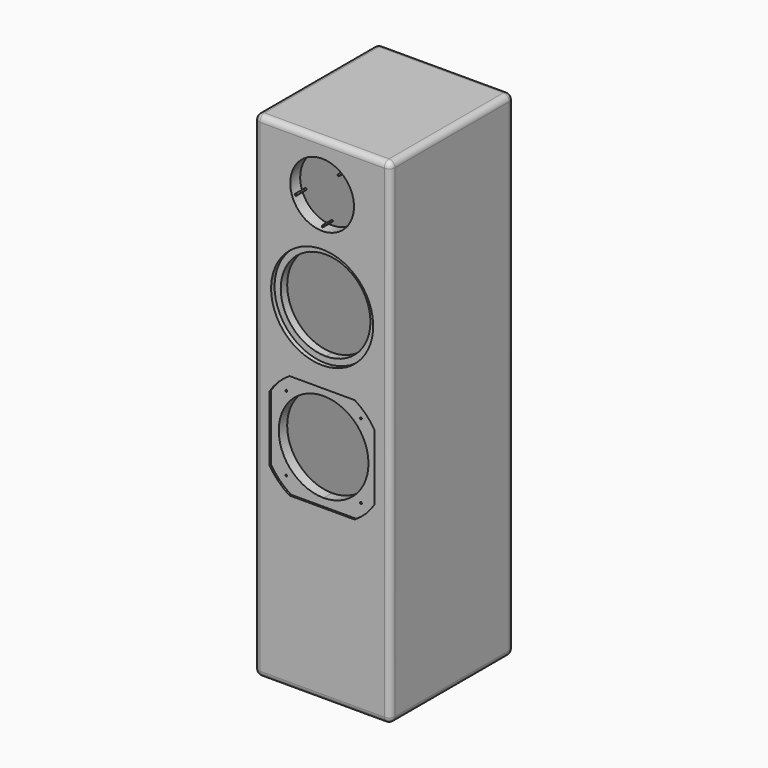
from build123d import *

# Parameters (mm, degrees)
F0_W     = 180
F0_H     = 210
F1_DEPTH = 20
F0_W_2   = 220
F0_H_2   = 250
F2_DEPTH = 800
F3_W     = 180
F3_H     = 210
F4_DEPTH = 20
F5_R     = 1.5
F6_DEPTH = 20
F7_DEPTH = 7
F8_DEPTH = 3
F9_R     = 9.5


with BuildPart() as f1:
    # F0 (on Top) → F1 (new body)
    with BuildSketch(Plane.XY):
        Rectangle(F0_W, F0_H)
    extrude(amount=F1_DEPTH)

    # F0 (on Top) → F2 (join)
    with BuildSketch(Plane.XY):
        Rectangle(F0_W_2, F0_H_2)
        Rectangle(F0_W, F0_H, mode=Mode.SUBTRACT)
    extrude(amount=F2_DEPTH)

    # F3 (on face) → F4 (join)
    with BuildSketch(Plane.XY.offset(800)):
        Rectangle(F3_W, F3_H)
    extrude(amount=-F4_DEPTH)

    # F5 (on face) → F6 (cut)
    with BuildSketch(Plane.XZ.offset(125)):
        with BuildLine():
            ThreePointArc((51.5, 720), (36.4159992311, 756.4159992311), (0, 771.5))
            Line((0, 771.5), (0, 765))
            ThreePointArc((0, 765), (13.1905408693, 763.023361463), (25.2222847872, 757.2670947367))
            ThreePointArc((25.2222847872, 757.2670947367), (26.9019571294, 757.8361628294), (27.9503363532, 756.4057647469))
            ThreePointArc((27.9503363532, 756.4057647469), (27.8730087425, 755.9303667321), (27.6489986565, 755.5039839073))
            ThreePointArc((27.6489986565, 755.5039839073), (40.4302172857, 739.7584799574), (45, 720))
            ThreePointArc((45, 720), (44.5571276947, 713.7021931119), (43.2372279289, 707.5283473019))
            ThreePointArc((43.2372279289, 707.5283473019), (44.0036790141, 706.9859955787), (44.2975432333, 706.0942352531))
            ThreePointArc((44.2975432333, 706.0942352531), (43.6690774316, 704.8734043307), (42.3103057118, 704.6755740541))
            ThreePointArc((42.3103057118, 704.6755740541), (26.4503363532, 683.5942352531), (1.4997916522, 675.025))
            ThreePointArc((1.4997916522, 675.025), (1.4999479121, 675.0125004341), (1.5, 675))
            ThreePointArc((1.5, 675), (1.0606601718, 673.9393398282), (0, 673.5))
            Line((0, 673.5), (0, 668.5))
            ThreePointArc((0, 668.5), (36.4159992311, 683.5840007689), (51.5, 720))
        make_face()
        with BuildLine():
            Line((0, 765), (0, 771.5))
            ThreePointArc((0, 771.5), (-51.5, 720), (0, 668.5))
            Line((0, 668.5), (0, 673.5))
            ThreePointArc((0, 673.5), (-1.0694624818, 673.9482158016), (-1.4997916522, 675.025))
            ThreePointArc((-1.4997916522, 675.025), (-26.4503363532, 683.5942352531), (-42.3103057118, 704.6755740541))
            ThreePointArc((-42.3103057118, 704.6755740541), (-44.2241280077, 705.6307097616), (-43.2372279289, 707.5283473019))
            ThreePointArc((-43.2372279289, 707.5283473019), (-42.7975432333, 733.9057647469), (-27.6489986565, 755.5039839073))
            ThreePointArc((-27.6489986565, 755.5039839073), (-27.3320142316, 757.6192902384), (-25.2222847872, 757.2670947367))
            ThreePointArc((-25.2222847872, 757.2670947367), (-13.1905408693, 763.023361463), (0, 765))
        make_face()
        with BuildLine():
            ThreePointArc((25.2222847872, 757.2670947367), (13.1905408693, 763.023361463), (0, 765))
            Line((0, 765), (0, 760))
            ThreePointArc((0, 760), (28.2842712475, 748.2842712475), (40, 720))
            ThreePointArc((40, 720), (28.2842712475, 691.7157287525), (0, 680))
            Line((0, 680), (0, 676.5))
            ThreePointArc((0, 676.5), (1.0517841984, 676.0694624818), (1.4997916522, 675.025))
            ThreePointArc((1.4997916522, 675.025), (26.4503363532, 683.5942352531), (42.3103057118, 704.6755740541))
            ThreePointArc((42.3103057118, 704.6755740541), (41.3709584588, 706.5577607447), (43.2372279289, 707.5283473019))
            ThreePointArc((43.2372279289, 707.5283473019), (44.5571276947, 713.7021931119), (45, 720))
            ThreePointArc((45, 720), (40.4302172857, 739.7584799574), (27.6489986565, 755.5039839073))
            ThreePointArc((27.6489986565, 755.5039839073), (25.5686584747, 755.1922392553), (25.2222847872, 757.2670947367))
        make_face()
        with BuildLine():
            Line((0, 760), (0, 765))
            ThreePointArc((0, 765), (-13.1905408693, 763.023361463), (-25.2222847872, 757.2670947367))
            ThreePointArc((-25.2222847872, 757.2670947367), (-25.0199382706, 756.8573855231), (-24.9503363532, 756.4057647469))
            ThreePointArc((-24.9503363532, 756.4057647469), (-25.9749383383, 754.9830923575), (-27.6489986565, 755.5039839073))
            ThreePointArc((-27.6489986565, 755.5039839073), (-42.7975432333, 733.9057647469), (-43.2372279289, 707.5283473019))
            ThreePointArc((-43.2372279289, 707.5283473019), (-41.9057829077, 707.3003710339), (-41.2975432333, 706.0942352531))
            ThreePointArc((-41.2975432333, 706.0942352531), (-41.5767123109, 705.2227010548), (-42.3103057118, 704.6755740541))
            ThreePointArc((-42.3103057118, 704.6755740541), (-26.4503363532, 683.5942352531), (-1.4997916522, 675.025))
            ThreePointArc((-1.4997916522, 675.025), (-1.0517841984, 676.0694624818), (0, 676.5))
            Line((0, 676.5), (0, 680))
            ThreePointArc((0, 680), (-40, 720), (0, 760))
        make_face()
        with BuildLine():
            ThreePointArc((40, 720), (28.2842712475, 748.2842712475), (0, 760))
            Line((0, 760), (0, 680))
            ThreePointArc((0, 680), (28.2842712475, 691.7157287525), (40, 720))
        make_face()
        with BuildLine():
            Line((0, 680), (0, 760))
            ThreePointArc((0, 760), (-40, 720), (0, 680))
        make_face()
        with BuildLine():
            ThreePointArc((-24.9503363532, 756.4057647469), (-25.0199382706, 756.8573855231), (-25.2222847872, 757.2670947367))
            ThreePointArc((-25.2222847872, 757.2670947367), (-26.4503363532, 756.4057647469), (-27.6489986565, 755.5039839073))
            ThreePointArc((-27.6489986565, 755.5039839073), (-25.9749383383, 754.9830923575), (-24.9503363532, 756.4057647469))
        make_face()
        with BuildLine():
            ThreePointArc((-27.6489986565, 755.5039839073), (-26.4503363532, 756.4057647469), (-25.2222847872, 757.2670947367))
            ThreePointArc((-25.2222847872, 757.2670947367), (-27.3320142316, 757.6192902384), (-27.6489986565, 755.5039839073))
        make_face()
        with BuildLine():
            ThreePointArc((-1.4997916522, 675.025), (-1.0694624818, 673.9482158016), (0, 673.5))
            Line((0, 673.5), (0, 675))
            ThreePointArc((0, 675), (-0.75, 675.0062504341), (-1.4997916522, 675.025))
        make_face()
        with BuildLine():
            ThreePointArc((-1.4997916522, 675.025), (-0.75, 675.0062504341), (0, 675))
            Line((0, 675), (0, 676.5))
            ThreePointArc((0, 676.5), (-1.0517841984, 676.0694624818), (-1.4997916522, 675.025))
        make_face()
        with BuildLine():
            ThreePointArc((72.5, 560), (51.265241636, 611.265241636), (0, 632.5))
            Line((0, 632.5), (0, 487.5))
            ThreePointArc((0, 487.5), (51.265241636, 508.734758364), (72.5, 560))
        make_face()
        with BuildLine():
            Line((0, 487.5), (0, 632.5))
            ThreePointArc((0, 632.5), (-72.5, 560), (0, 487.5))
        make_face()
        with BuildLine():
            ThreePointArc((44.2975432333, 706.0942352531), (44.0036790141, 706.9859955787), (43.2372279289, 707.5283473019))
            ThreePointArc((43.2372279289, 707.5283473019), (42.7975432333, 706.0942352531), (42.3103057118, 704.6755740541))
            ThreePointArc((42.3103057118, 704.6755740541), (43.6690774316, 704.8734043307), (44.2975432333, 706.0942352531))
        make_face()
        with BuildLine():
            ThreePointArc((42.3103057118, 704.6755740541), (42.7975432333, 706.0942352531), (43.2372279289, 707.5283473019))
            ThreePointArc((43.2372279289, 707.5283473019), (41.3709584588, 706.5577607447), (42.3103057118, 704.6755740541))
        make_face()
        with BuildLine():
            ThreePointArc((0, 432.5), (-72.5, 360), (0, 287.5))
            Line((0, 287.5), (0, 432.5))
        make_face()
        with BuildLine():
            Line((0, 432.5), (0, 287.5))
            ThreePointArc((0, 287.5), (51.265241636, 308.734758364), (72.5, 360))
            ThreePointArc((72.5, 360), (51.265241636, 411.265241636), (0, 432.5))
        make_face()
        with Locations((-60.2813602239, 420.2813602239)):
            Circle(F5_R)
        with Locations((-60.2813602239, 299.7186397761)):
            Circle(F5_R)
        with Locations((60.2813602239, 299.7186397761)):
            Circle(F5_R)
        with Locations((60.2813602239, 420.2813602239)):
            Circle(F5_R)
    extrude(amount=-F6_DEPTH, mode=Mode.SUBTRACT)

    # F5 (on face) → F7 (cut)
    with BuildSketch(Plane.XZ.offset(125)):
        with BuildLine():
            Line((0, 632.5), (0, 642.5))
            ThreePointArc((0, 642.5), (-82.5, 560), (0, 477.5))
            Line((0, 477.5), (0, 487.5))
            ThreePointArc((0, 487.5), (-72.5, 560), (0, 632.5))
        make_face()
        with BuildLine():
            ThreePointArc((82.5, 560), (58.3363094479, 618.3363094479), (0, 642.5))
            Line((0, 642.5), (0, 632.5))
            ThreePointArc((0, 632.5), (51.265241636, 611.265241636), (72.5, 560))
            ThreePointArc((72.5, 560), (51.265241636, 508.734758364), (0, 487.5))
            Line((0, 487.5), (0, 477.5))
            ThreePointArc((0, 477.5), (58.3363094479, 501.6636905521), (82.5, 560))
        make_face()
    extrude(amount=-F7_DEPTH, mode=Mode.SUBTRACT)

    # F5 (on face) → F8 (cut)
    with BuildSketch(Plane.XZ.offset(125)):
        with BuildLine():
            Line((-52.6782687643, 275), (0, 275))
            Line((0, 275), (0, 287.5))
            ThreePointArc((0, 287.5), (-72.5, 360), (0, 432.5))
            Line((0, 432.5), (0, 445))
            Line((0, 445), (-52.6782687643, 445))
            ThreePointArc((-52.6782687643, 445), (-70.7106781187, 430.7106781187), (-85, 412.6782687643))
            Line((-85, 412.6782687643), (-85, 307.3217312357))
            ThreePointArc((-85, 307.3217312357), (-70.7106781187, 289.2893218813), (-52.6782687643, 275))
        make_face()
        with Locations((-60.2813602239, 299.7186397761)):
            Circle(F5_R, mode=Mode.SUBTRACT)
        with Locations((-60.2813602239, 420.2813602239)):
            Circle(F5_R, mode=Mode.SUBTRACT)
        with BuildLine():
            Line((0, 287.5), (0, 275))
            Line((0, 275), (52.6782687643, 275))
            ThreePointArc((52.6782687643, 275), (70.7106781187, 289.2893218813), (85, 307.3217312357))
            Line((85, 307.3217312357), (85, 412.6782687643))
            ThreePointArc((85, 412.6782687643), (70.7106781187, 430.7106781187), (52.6782687643, 445))
            Line((52.6782687643, 445), (0, 445))
            Line((0, 445), (0, 432.5))
            ThreePointArc((0, 432.5), (51.265241636, 411.265241636), (72.5, 360))
            ThreePointArc((72.5, 360), (51.265241636, 308.734758364), (0, 287.5))
        make_face()
        with Locations((60.2813602239, 299.7186397761)):
            Circle(F5_R, mode=Mode.SUBTRACT)
        with Locations((60.2813602239, 420.2813602239)):
            Circle(F5_R, mode=Mode.SUBTRACT)
        with BuildLine():
            Line((0, 765), (0, 771.5))
            ThreePointArc((0, 771.5), (-51.5, 720), (0, 668.5))
            Line((0, 668.5), (0, 673.5))
            ThreePointArc((0, 673.5), (-1.0694624818, 673.9482158016), (-1.4997916522, 675.025))
            ThreePointArc((-1.4997916522, 675.025), (-26.4503363532, 683.5942352531), (-42.3103057118, 704.6755740541))
            ThreePointArc((-42.3103057118, 704.6755740541), (-44.2241280077, 705.6307097616), (-43.2372279289, 707.5283473019))
            ThreePointArc((-43.2372279289, 707.5283473019), (-42.7975432333, 733.9057647469), (-27.6489986565, 755.5039839073))
            ThreePointArc((-27.6489986565, 755.5039839073), (-27.3320142316, 757.6192902384), (-25.2222847872, 757.2670947367))
            ThreePointArc((-25.2222847872, 757.2670947367), (-13.1905408693, 763.023361463), (0, 765))
        make_face()
        with BuildLine():
            ThreePointArc((51.5, 720), (36.4159992311, 756.4159992311), (0, 771.5))
            Line((0, 771.5), (0, 765))
            ThreePointArc((0, 765), (13.1905408693, 763.023361463), (25.2222847872, 757.2670947367))
            ThreePointArc((25.2222847872, 757.2670947367), (26.9019571294, 757.8361628294), (27.9503363532, 756.4057647469))
            ThreePointArc((27.9503363532, 756.4057647469), (27.8730087425, 755.9303667321), (27.6489986565, 755.5039839073))
            ThreePointArc((27.6489986565, 755.5039839073), (40.4302172857, 739.7584799574), (45, 720))
            ThreePointArc((45, 720), (44.5571276947, 713.7021931119), (43.2372279289, 707.5283473019))
            ThreePointArc((43.2372279289, 707.5283473019), (44.0036790141, 706.9859955787), (44.2975432333, 706.0942352531))
            ThreePointArc((44.2975432333, 706.0942352531), (43.6690774316, 704.8734043307), (42.3103057118, 704.6755740541))
            ThreePointArc((42.3103057118, 704.6755740541), (26.4503363532, 683.5942352531), (1.4997916522, 675.025))
            ThreePointArc((1.4997916522, 675.025), (1.4999479121, 675.0125004341), (1.5, 675))
            ThreePointArc((1.5, 675), (1.0606601718, 673.9393398282), (0, 673.5))
            Line((0, 673.5), (0, 668.5))
            ThreePointArc((0, 668.5), (36.4159992311, 683.5840007689), (51.5, 720))
        make_face()
        with BuildLine():
            Line((0, 760), (0, 765))
            ThreePointArc((0, 765), (-13.1905408693, 763.023361463), (-25.2222847872, 757.2670947367))
            ThreePointArc((-25.2222847872, 757.2670947367), (-25.0199382706, 756.8573855231), (-24.9503363532, 756.4057647469))
            ThreePointArc((-24.9503363532, 756.4057647469), (-25.9749383383, 754.9830923575), (-27.6489986565, 755.5039839073))
            ThreePointArc((-27.6489986565, 755.5039839073), (-42.7975432333, 733.9057647469), (-43.2372279289, 707.5283473019))
            ThreePointArc((-43.2372279289, 707.5283473019), (-41.9057829077, 707.3003710339), (-41.2975432333, 706.0942352531))
            ThreePointArc((-41.2975432333, 706.0942352531), (-41.5767123109, 705.2227010548), (-42.3103057118, 704.6755740541))
            ThreePointArc((-42.3103057118, 704.6755740541), (-26.4503363532, 683.5942352531), (-1.4997916522, 675.025))
            ThreePointArc((-1.4997916522, 675.025), (-1.0517841984, 676.0694624818), (0, 676.5))
            Line((0, 676.5), (0, 680))
            ThreePointArc((0, 680), (-40, 720), (0, 760))
        make_face()
        with BuildLine():
            ThreePointArc((25.2222847872, 757.2670947367), (13.1905408693, 763.023361463), (0, 765))
            Line((0, 765), (0, 760))
            ThreePointArc((0, 760), (28.2842712475, 748.2842712475), (40, 720))
            ThreePointArc((40, 720), (28.2842712475, 691.7157287525), (0, 680))
            Line((0, 680), (0, 676.5))
            ThreePointArc((0, 676.5), (1.0517841984, 676.0694624818), (1.4997916522, 675.025))
            ThreePointArc((1.4997916522, 675.025), (26.4503363532, 683.5942352531), (42.3103057118, 704.6755740541))
            ThreePointArc((42.3103057118, 704.6755740541), (41.3709584588, 706.5577607447), (43.2372279289, 707.5283473019))
            ThreePointArc((43.2372279289, 707.5283473019), (44.5571276947, 713.7021931119), (45, 720))
            ThreePointArc((45, 720), (40.4302172857, 739.7584799574), (27.6489986565, 755.5039839073))
            ThreePointArc((27.6489986565, 755.5039839073), (25.5686584747, 755.1922392553), (25.2222847872, 757.2670947367))
        make_face()
    extrude(amount=-F8_DEPTH, mode=Mode.SUBTRACT)

    # F9
    f9_edges = [f1.edges().sort_by_distance(p)[0] for p in [
        (0, -125, 800),
        (110, 0, 800),
        (110, -125, 400),
        (110, 125, 400),
        (0, 125, 800),
        (-110, 0, 800),
        (-110, -125, 400),
        (0, -125, 0),
        (-110, 125, 400),
        (-110, 0, 0),
        (110, 0, 0),
        (0, 125, 0),
    ]]
    fillet(f9_edges, radius=F9_R)


solid = f1.part
